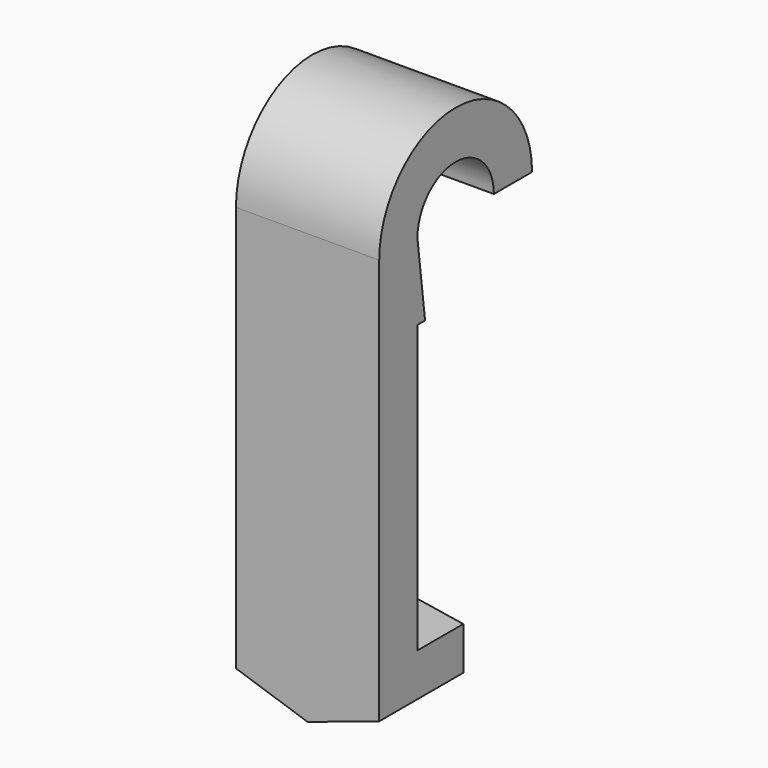
from build123d import *

# Parameters (mm, degrees)
F0_W        = 15
F0_H        = 5
F1_DEPTH    = 38
F2_W        = 15
F2_H        = 5
F3_DEPTH    = 7
F4_T1_DEPTH = 50.0054850444
F1_FACE1_W  = 15
F1_FACE1_H  = 5
F8_DEPTH    = 15


# Not quite as in the source:
# - a fillet or chamfer that OpenCascade refuses, or shapes differently, is made with other operations: its cross-section is extruded or revolved along the edge and cut away or added


with BuildPart() as f1:
    # F0 (on Top) → F1 (new body)
    with BuildSketch(Plane.XY):
        with Locations((0, 2.5)):
            Rectangle(F0_W, F0_H)
    extrude(amount=F1_DEPTH)

    # F2 (on face) → F3 (join)
    with BuildSketch(Plane(origin=(0, 0, 0), x_dir=(1, 0, 0), z_dir=(0, 0, -1))):
        Polygon((7.5, -10), (7.5, -5), (-7.5, -5), (-7.5, -10), (-7.5, -11), (0, -12.5), (7.5, -11), align=None)
        with Locations((0, -2.5)):
            Rectangle(F2_W, F2_H)
    extrude(amount=F3_DEPTH)

    # F4: chamfer of 2.5 x 7.5152772587 on 2 edges, made by hand

    # F4_s2 → F4_t1 (cut)
    with BuildSketch(Plane.XZ.offset(-30.5027425222)):
        Polygon((0.0152772587, -7), (-7.5, -4.5), (-7.5, -7), align=None)
        Polygon((-0.0152772587, -7), (7.5, -4.5), (7.5, -7), align=None)
    extrude(amount=F4_T1_DEPTH, mode=Mode.SUBTRACT)

    # F6: sweep along a path in F5
    with BuildLine(Plane.YZ.offset(7.5)) as f6_path:
        ThreePointArc((17.5, 38), (10, 45.5), (2.5, 38))
    # F1_face1 (on face) → F6 (sweep)
    with BuildSketch(Plane(origin=(0, 2.5, 38), x_dir=(1, 0, 0), z_dir=(0, 0, 1))):
        Rectangle(F1_FACE1_W, F1_FACE1_H)
    sweep(path=f6_path.line)

    # F7 (on face) → F8 (join)
    with BuildSketch(Plane.YZ.offset(7.5)):
        Polygon((6, 30), (5, 38), (5, 30), align=None)
    extrude(amount=-F8_DEPTH)


solid = f1.part
